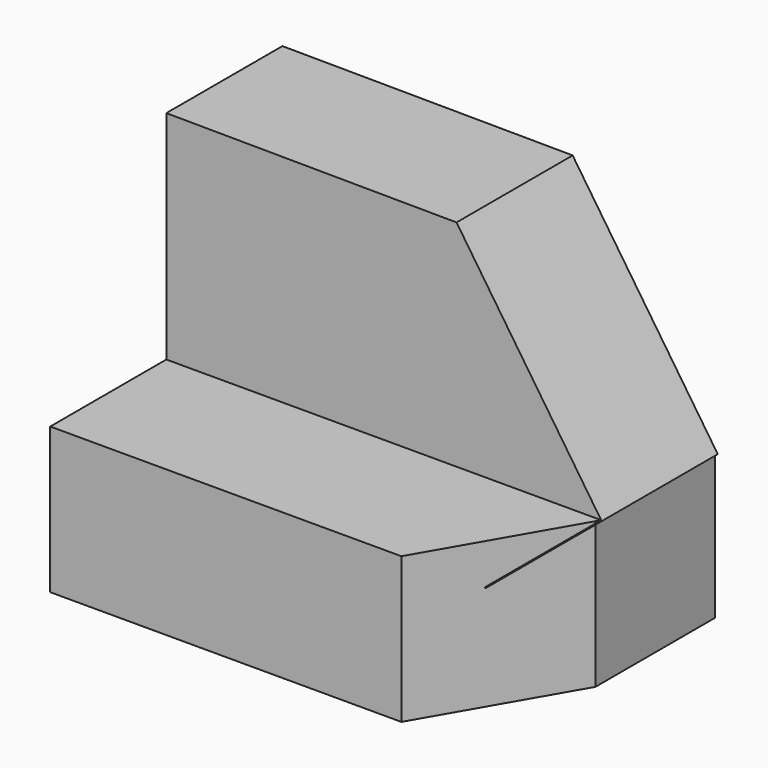
from build123d import *

# Parameters (mm, degrees)
F1_DEPTH  = 25.4
F3_DEPTH  = 82
F1_FACE_W = 25.4
F1_FACE_H = 31.75
F4_DEPTH  = 25.4
F5_W      = 12.7
F5_H      = 18.9845859185
F6_DEPTH  = 38.101
F8_DEPTH  = 25.4
F9_W      = 25.4
F9_H      = 12.7
F10_DEPTH = 0.254


# Not quite as in the source:
# - an extrude ends at something that could not be found from the text; its depth is read off the source's solid


with BuildPart() as f1:
    # F0 (on Front) → F1 (new body)
    with BuildSketch(Plane.XZ):
        Polygon((25.3994814964, 31.5877048481), (0, 31.75), (0, 0), (38.1, 0), (38.1, 12.7), align=None)
    extrude(amount=F1_DEPTH)

    # F2 (on Right) → F3 (cut, through all)
    with BuildSketch(Plane.YZ):
        Polygon((-12.9239121452, 31.9192558527), (-25.5880542099, 31.9192558527), (-25.4064481705, 12.6858642325), (-12.9239121452, 12.6858642325), align=None)
    extrude(amount=-F3_DEPTH, mode=Mode.SUBTRACT)

    # F2 (on Right) + F1_face (on face) → F4 (cut)
    with BuildSketch(Plane.YZ):
        Polygon((-12.9239121452, 31.9192558527), (-25.5880542099, 31.9192558527), (-25.4064481705, 12.6858642325), (-12.9239121452, 12.6858642325), align=None)
    with BuildSketch(Plane(origin=(0, -12.7, 15.875), x_dir=(0, -1, 0), z_dir=(-1, 0, 0))):
        Rectangle(F1_FACE_W, F1_FACE_H)
    extrude(amount=-F4_DEPTH, dir=(1, 0, 0), mode=Mode.SUBTRACT)

    # F5 (on face) → F6 (cut, through all)
    with BuildSketch(Plane(origin=(0, 0, 0), x_dir=(0, -1, 0), z_dir=(-1, 0, 0))):
        with Locations((19.05, 22.2577070408)):
            Rectangle(F5_W, F5_H)
    extrude(amount=-F6_DEPTH, mode=Mode.SUBTRACT)

    # F7 (on face) → F8 (cut)
    with BuildSketch(Plane.XY.offset(12.7654140815)):
        Polygon((38.056014097, -25.4), (38.056014097, -12.7), (30.7297278196, -25.4), align=None)
    extrude(amount=-F8_DEPTH, mode=Mode.SUBTRACT)

    # F9 (on face) → F10 (cut)
    with BuildSketch(Plane.YZ.offset(38.1)):
        with Locations((-12.7, 6.35)):
            Rectangle(F9_W, F9_H)
    extrude(amount=-F10_DEPTH, mode=Mode.SUBTRACT)


solid = f1.part
